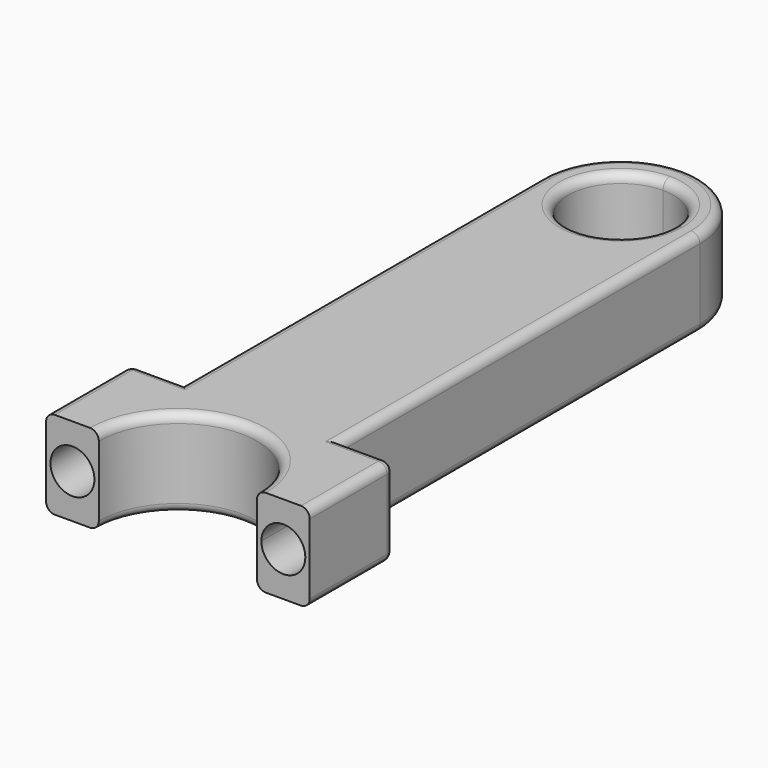
from build123d import *

# Parameters (mm, degrees)
F1_DEPTH = 5
F2_R     = 4.49999
F3_R     = 0.5
F5_DEPTH = 5


# Not quite as in the source:
# - a fillet or chamfer is up to 0.001 mm smaller than in the source, because OpenCascade refuses the exact size
# - a feature names something its author has since deleted; it is built from what else it names


with BuildPart() as f1:
    # F0 (on Top) → F1 (new body)
    with BuildSketch(Plane.XY):
        with BuildLine():
            Line((4.5, -14.8228148893), (-4.5, -14.8228148893))
            Line((-4.5, -14.8228148893), (-7.5, -14.8228148893))
            Line((-7.5, -14.8228148893), (-7.5, -20.8228148893))
            Line((-7.5, -20.8228148893), (-4.5, -20.8228148893))
            ThreePointArc((-4.5, -20.8228148893), (0, -16.3228148893), (4.5, -20.8228148893))
            Line((4.5, -20.8228148893), (7.5, -20.8228148893))
            Line((7.5, -20.8228148893), (7.5, -14.8228148893))
            Line((7.5, -14.8228148893), (4.5, -14.8228148893))
        make_face()
        Polygon((0, 15.1771851107), (-4.5, 15.1771851107), (-4.5, -14.8228148893), (4.5, -14.8228148893), (4.5, 15.1771851107), align=None)
        with BuildLine():
            ThreePointArc((3, 10.6771851107), (-2.1213203436, 8.5558647672), (0, 13.6771851107))
            ThreePointArc((0, 13.6771851107), (2.1213203436, 12.7985054543), (3, 10.6771851107))
        make_face(mode=Mode.SUBTRACT)
    extrude(amount=F1_DEPTH)

    # F2 (radius 4.5 in the source; OpenCascade refuses exactly that, so slightly less here)
    f2_edges = [f1.edges().sort_by_distance(p)[0] for p in [
        (4.5, 15.177185, 2.5),
        (-4.5, 15.177185, 2.5),
    ]]
    fillet(f2_edges, radius=F2_R)

    # F3
    f3_edges = [f1.edges().sort_by_distance(p)[0] for p in [
        (-4.5, -2.07281, 5),
        (-4.5, -2.07281, 0),
        (-6, -14.822815, 5),
        (-6, -14.822815, 0),
        (-7.5, -14.822815, 2.5),
        (7.5, -14.822815, 2.5),
        (6, -14.822815, 0),
        (6, -14.822815, 5),
        (-7.5, -17.822815, 0),
        (-7.5, -17.822815, 5),
        (7.5, -17.822815, 5),
        (7.5, -17.822815, 0),
        (-3, 10.677185, 5),
        (-3, 10.677185, 0),
        (0, -16.322815, 5),
        (0, -16.322815, 0),
        (4.5, -2.07281, 0),
        (4.5, -2.07281, 5),
        (3.181983, 13.859169, 0),
        (0, 15.177185, 0),
        (-3.181983, 13.859169, 0),
        (3.181983, 13.859169, 5),
        (0, 15.177185, 5),
        (-3.181983, 13.859169, 5),
    ]]
    fillet(f3_edges, radius=F3_R)

    # F4 (on face) → F5 (cut)
    with BuildSketch(Plane.XZ.offset(20.8228148893)):
        with BuildLine():
            ThreePointArc((7.25, 2.5), (6.8838834765, 3.3838834765), (6, 3.75))
            Line((6, 3.75), (6, 2.5))
            Line((6, 2.5), (4.75, 2.5))
            ThreePointArc((4.75, 2.5), (6, 1.25), (7.25, 2.5))
        make_face()
        with BuildLine():
            Line((6, 2.5), (6, 3.75))
            ThreePointArc((6, 3.75), (5.1161165235, 3.3838834765), (4.75, 2.5))
            Line((4.75, 2.5), (6, 2.5))
        make_face()
        with BuildLine():
            Line((-6, 2.5), (-6, 3.75))
            ThreePointArc((-6, 3.75), (-6.8838834765, 1.6161165235), (-4.75, 2.5))
            Line((-4.75, 2.5), (-6, 2.5))
        make_face()
        with BuildLine():
            ThreePointArc((-4.75, 2.5), (-5.1161165235, 3.3838834765), (-6, 3.75))
            Line((-6, 3.75), (-6, 2.5))
            Line((-6, 2.5), (-4.75, 2.5))
        make_face()
    extrude(amount=-F5_DEPTH, mode=Mode.SUBTRACT)


solid = f1.part
